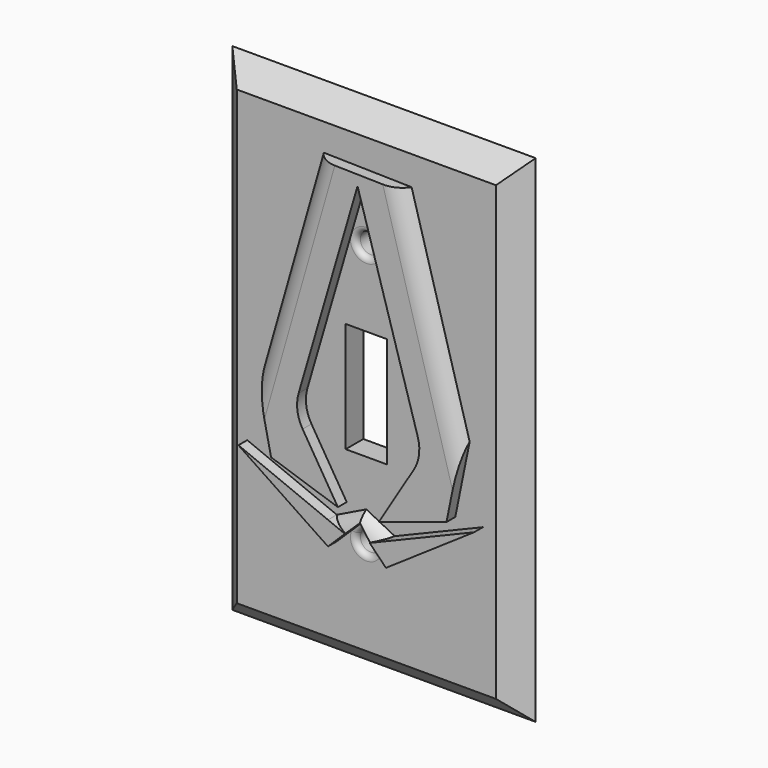
from build123d import *

# Parameters (mm, degrees)
F0_W         = 69.85
F0_H         = 114.3
F0_R         = 2.3876
F0_W_2       = 9.525
F0_H_2       = 25.4
F1_DEPTH     = 5.08
F2_SIZE      = 5.07999
F4_DEPTH     = 2.54
F5_T1_DEPTH  = 71.5966436916
F5_T3_DEPTH  = 71.1214770669
F5_T8_DEPTH  = 29.3324993846
F5_T14_DEPTH = 29.5628780991
F6_R         = 1.27


# Not quite as in the source:
# - a fillet or chamfer that OpenCascade refuses, or shapes differently, is made with other operations: its cross-section is extruded or revolved along the edge and cut away or added
# - a fillet or chamfer is up to 0.001 mm smaller than in the source, because OpenCascade refuses the exact size


with BuildPart() as f1:
    # F0 (on Front) → F1 (new body)
    with BuildSketch(Plane.XZ):
        Rectangle(F0_W, F0_H)
        with Locations((0, -30.1625)):
            Circle(F0_R, mode=Mode.SUBTRACT)
        Rectangle(F0_W_2, F0_H_2, mode=Mode.SUBTRACT)
        with Locations((0, 30.1625)):
            Circle(F0_R, mode=Mode.SUBTRACT)
    extrude(amount=F1_DEPTH)

    # F2 (size 5.08 in the source; OpenCascade refuses exactly that, so slightly less here)
    f2_edges = [f1.edges().sort_by_distance(p)[0] for p in [
        (0, -5.08, 57.15),
        (34.925, -5.08, 0),
        (0, -5.08, -57.15),
        (-34.925, -5.08, 0),
    ]]
    chamfer(f2_edges, length=F2_SIZE)

    # F3 (on face) → F4 (join)
    with BuildSketch(Plane.XZ.offset(5.08)):
        with BuildLine():
            Line((10.4210752899, 45.360866621), (-9.7815324138, 45.7814973))
            Line((-9.7815324138, 45.7814973), (-23.4081424498, -1.9095465541))
            Line((-23.4081424498, -1.9095465541), (-19.9071371743, -18.2295814157))
            Line((-19.9071371743, -18.2295814157), (-4.5221770743, -23.345419034))
            Line((-4.5221770743, -23.345419034), (-12.6387388145, -10.1591296217))
            ThreePointArc((-12.6387388145, -10.1591296217), (-13.8432881685, -6.7829644544), (-13.5732137506, -3.2085427961))
            Line((-13.5732137506, -3.2085427961), (0, 43.2110093534))
            Line((0, 43.2110093534), (13.8653954743, -3.0792306258))
            ThreePointArc((13.8653954743, -3.0792306258), (14.1574638309, -6.6629312481), (12.9648391888, -10.0549602188))
            Line((12.9648391888, -10.0549602188), (4.856493974, -23.345419034))
            Line((4.856493974, -23.345419034), (20.4867540311, -18.2295814157))
            Line((20.4867540311, -18.2295814157), (23.789614439, -1.9095465541))
            Line((23.789614439, -1.9095465541), (10.4210752899, 45.360866621))
        make_face()
        Polygon((6.5450641223, -26.6576724823), (0, -23.345419034), (-6.802264601, -26.6576724823), (-27.4259783328, -18.2295814157), (-6.802264601, -32.0519991219), (0, -25.3795739263), (6.5450641223, -32.0519991219), (26.8477257341, -18.2295814157), align=None)
    extrude(amount=F4_DEPTH)

    # F5: fillet of radius 5.08 on 4 edges, made by hand

    # F5_s2 → F5_t1 (cut)
    with BuildSketch(Plane(origin=(14.3770362631, 0, 50.317420481), x_dir=(0, 1, 0), z_dir=(-0.2747322653, 0, -0.9615207655))):
        with BuildLine():
            ThreePointArc((-5.08, -21.9828009958), (-6.9394090512, -20.1233919446), (-7.62, -17.5833919446))
            Line((-7.62, -17.5833919446), (-7.62, -21.9828009958))
            Line((-7.62, -21.9828009958), (-5.08, -21.9828009958))
        make_face()
    extrude(amount=F5_T1_DEPTH, mode=Mode.SUBTRACT)

    # F5_s4 → F5_t3 (cut)
    with BuildSketch(Plane(origin=(5.2549558521, 0, -18.5812325171), x_dir=(0, 1, 0), z_dir=(-0.27213626, 0, 0.9622587261))):
        with BuildLine():
            ThreePointArc((-5.08, -22.3721072272), (-6.9394090512, -20.5126981759), (-7.62, -17.9726981759))
            Line((-7.62, -17.9726981759), (-7.62, -22.3721072272))
            Line((-7.62, -22.3721072272), (-5.08, -22.3721072272))
        make_face()
    extrude(amount=F5_T3_DEPTH, mode=Mode.SUBTRACT)


with BuildPart() as f5_tool6:
    # F5_s7 → F5_t8 (new body)
    with BuildSketch(Plane(origin=(25.7640738936, 0, -13.0383967217), x_dir=(0, 1, 0), z_dir=(-0.8922507056, 0, 0.4515403396))):
        with BuildLine():
            ThreePointArc((-5.08, 20.8299666066), (-6.9394090512, 22.6893756578), (-7.62, 25.2293756578))
            Line((-7.62, 25.2293756578), (-7.62, 20.8299666066))
            Line((-7.62, 20.8299666066), (-5.08, 20.8299666066))
        make_face()
    extrude(amount=F5_T8_DEPTH)

    split(bisect_by=Plane(origin=(10.401612722, 0, -25.0567324961), x_dir=(0, 1, 0), z_dir=(-0.3833998348, 0, 0.9235824634)), keep=Keep.TOP)

    split(bisect_by=Plane(origin=(9.1889369632, 0, -18.8710138282), x_dir=(0, 1, 0), z_dir=(0.4377909897, 0, -0.8990767761)), keep=Keep.TOP)


with BuildPart() as f1_1:
    add(f1.part)

    # F5_t5: cut F5_tool6
    add(f5_tool6.part, mode=Mode.SUBTRACT)


with BuildPart() as f5_tool12:
    # F5_s13 → F5_t14 (new body)
    with BuildSketch(Plane(origin=(0.6995793032, 0, 0.3406489008), x_dir=(0, 1, 0), z_dir=(-0.8990767761, 0, -0.4377909897))):
        with BuildLine():
            ThreePointArc((-5.08, 20.9893240819), (-6.9394090512, 22.8487331332), (-7.62, 25.3887331332))
            Line((-7.62, 25.3887331332), (-7.62, 20.9893240819))
            Line((-7.62, 20.9893240819), (-5.08, 20.9893240819))
        make_face()
    extrude(amount=F5_T14_DEPTH)

    split(bisect_by=Plane(origin=(-9.4055701954, 0, -18.5855524032), x_dir=(0, 1, 0), z_dir=(-0.4515403396, 0, -0.8922507056)), keep=Keep.TOP)

    split(bisect_by=Plane(origin=(-10.3083950149, 0, -25.2248565112), x_dir=(0, 1, 0), z_dir=(0.3782912807, 0, 0.9256866138)), keep=Keep.TOP)


with BuildPart() as f1_2:
    add(f1_1.part)

    # F5_t11: cut F5_tool12
    add(f5_tool12.part, mode=Mode.SUBTRACT)

    # F6
    f6_edges = [f1_2.edges().sort_by_distance(p)[0] for p in [
        (-2.3876, -5.08, 30.1625),
        (-2.3876, -5.08, -30.1625),
    ]]
    fillet(f6_edges, radius=F6_R)


solid = f1_2.part
